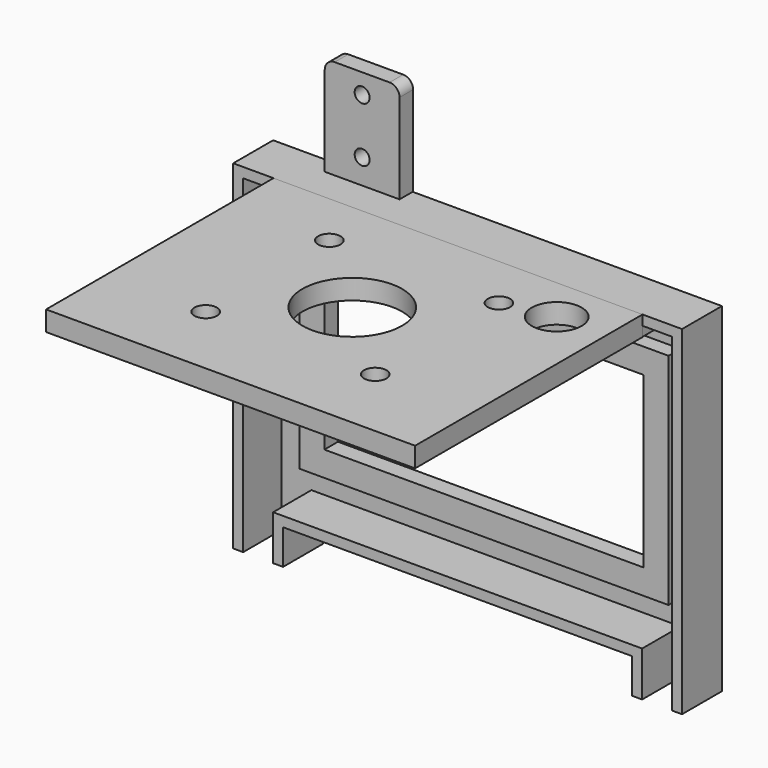
from build123d import *

# Parameters (mm, degrees)
F2_DEPTH = 10
F4_W     = 74
F4_H     = 57
F4_R     = 2.25
F4_R_2   = 10
F4_R_3   = 5
F5_DEPTH = 4
F0_W     = 74
F0_H     = 44
F6_DEPTH = 0.4
F0_W_2   = 64
F0_H_2   = 34
F7_DEPTH = 3.4
F8_R     = 1.5
F9_DEPTH = 3.4


with BuildPart() as f2:
    # F0 (on Front) → F2 (new body)
    with BuildSketch(Plane.XZ):
        Polygon((0, 2), (0, -64), (2, -64), (2, 4), (-88, 4), (-88, -64), (-86, -64), (-86, 2), (-80, 2), (-80, 0), (-6, 0), (-6, 2), align=None)
    extrude(amount=F2_DEPTH)


with BuildPart() as f2b:
    # F0 (on Front) → F2, piece 2 (new body)
    with BuildSketch(Plane.XZ):
        Polygon((-6, -64), (-6, -55), (-80, -55), (-80, -64), (-78, -64), (-78, -57), (-8, -57), (-8, -64), align=None)
    extrude(amount=F2_DEPTH)

    # F0 (on Front) → F6 (join)
    with BuildSketch(Plane.XZ):
        Polygon((-80, -55), (-6, -55), (-6, -64), (0, -64), (0, 2), (-6, 2), (-6, 0), (-80, 0), (-80, 2), (-86, 2), (-86, -64), (-80, -64), align=None)
        with Locations((-43, -28)):
            Rectangle(F0_W, F0_H, mode=Mode.SUBTRACT)
    extrude(amount=F6_DEPTH)

    # F0 (on Front) → F7 (join)
    with BuildSketch(Plane.XZ):
        with Locations((-43, -28)):
            Rectangle(F0_W, F0_H)
        with Locations((-43, -28)):
            Rectangle(F0_W_2, F0_H_2, mode=Mode.SUBTRACT)
    extrude(amount=F7_DEPTH)


with BuildPart() as f5:
    # F4 (on face) → F5 (new body, through all)
    with BuildSketch(Plane.XY.offset(4)):
        with Locations((-42.927035287, -38.5)):
            Rectangle(F4_W, F4_H)
        with Locations((-59.927035287, -52)):
            Circle(F4_R, mode=Mode.SUBTRACT)
        with Locations((-25.927035287, -52)):
            Circle(F4_R, mode=Mode.SUBTRACT)
        with Locations((-42.927035287, -36.5)):
            Circle(F4_R_2, mode=Mode.SUBTRACT)
        with Locations((-59.927035287, -21)):
            Circle(F4_R, mode=Mode.SUBTRACT)
        with Locations((-25.927035287, -21)):
            Circle(F4_R, mode=Mode.SUBTRACT)
        with Locations((-15.927035287, -19)):
            Circle(F4_R_3, mode=Mode.SUBTRACT)
    extrude(amount=-F5_DEPTH)


with BuildPart() as f9:
    # F8 (on Front) → F9 (new body)
    with BuildSketch(Plane.XZ):
        with BuildLine():
            Line((-74.927035287, 4.0744631551), (-59.927035287, 4.0744631551))
            Line((-59.927035287, 4.0744631551), (-59.927035287, 22.0744631551))
            ThreePointArc((-59.927035287, 22.0744631551), (-60.5128217246, 23.4886767175), (-61.927035287, 24.0744631551))
            Line((-61.927035287, 24.0744631551), (-72.927035287, 24.0744631551))
            ThreePointArc((-72.927035287, 24.0744631551), (-74.3412488494, 23.4886767175), (-74.927035287, 22.0744631551))
            Line((-74.927035287, 22.0744631551), (-74.927035287, 4.0744631551))
        make_face()
        with Locations((-67.427035287, 9.0744631551)):
            Circle(F8_R, mode=Mode.SUBTRACT)
        with Locations((-67.427035287, 20.0744631551)):
            Circle(F8_R, mode=Mode.SUBTRACT)
    extrude(amount=F9_DEPTH)


solid = Compound([f2.part, f2b.part, f5.part, f9.part])
